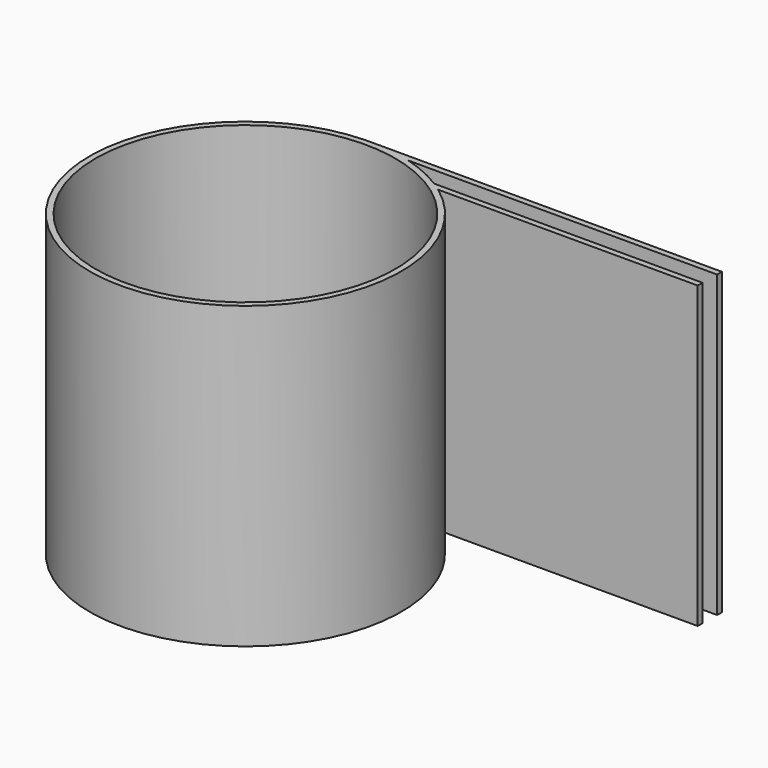
from build123d import *

# Parameters (mm, degrees)
F1_DEPTH = 50
F3_D     = 50


# Not quite as in the source:
# - the program builds the solid bodies; features that only make, move or delete a surface that nothing else refers to are left out


with BuildPart() as f1:
    # F0 (on Top) → F1 (new body)
    with BuildSketch(Plane.XY):
        with BuildLine():
            Line((49.3272994906, 40.4565469784), (-10.1727005094, 40.4565469784))
            ThreePointArc((-10.1727005094, 40.4565469784), (-17.0425953064, -10.3691748199), (5.9889720653, 35.4565423621))
            Line((5.9889720653, 35.4565423621), (49.2908384362, 35.4565423621))
            Line((49.2908384362, 35.4565423621), (49.2908384362, 36.4565423621))
            Line((49.2908384362, 36.4565423621), (4.5184440125, 36.4565423621))
            ThreePointArc((4.5184440125, 36.4565423621), (1.2797957907, 38.1934060872), (-2.1713849513, 39.4562953896))
            Line((-2.1713849513, 39.4562953896), (49.3272994906, 39.4562953896))
            Line((49.3272994906, 39.4562953896), (49.3272994906, 40.4565469784))
        make_face()
        with BuildLine():
            ThreePointArc((-10.1647124973, 39.4562953896), (8.0319806239, 32.4298558016), (15.6417905006, 14.4693077177))
            ThreePointArc((15.6417905006, 14.4693077177), (-26.7483996228, -3.4912403662), (-10.1647124973, 39.4562953896))
        make_face(mode=Mode.SUBTRACT)
        with BuildLine():
            ThreePointArc((-10.1647124973, 39.4562953896), (-26.7483996228, -3.4912403662), (15.6417905006, 14.4693077177))
            ThreePointArc((15.6417905006, 14.4693077177), (8.0319806239, 32.4298558016), (-10.1647124973, 39.4562953896))
        make_face()
    extrude(amount=F1_DEPTH)

    # F3 (through all)
    with Locations(Plane(origin=(0, 0, 0), x_dir=(1, 0, 0), z_dir=(0, 0, -1))):
        with Locations((-9.3582094994, -14.4693077177)):
            Hole(F3_D / 2)


solid = f1.part
